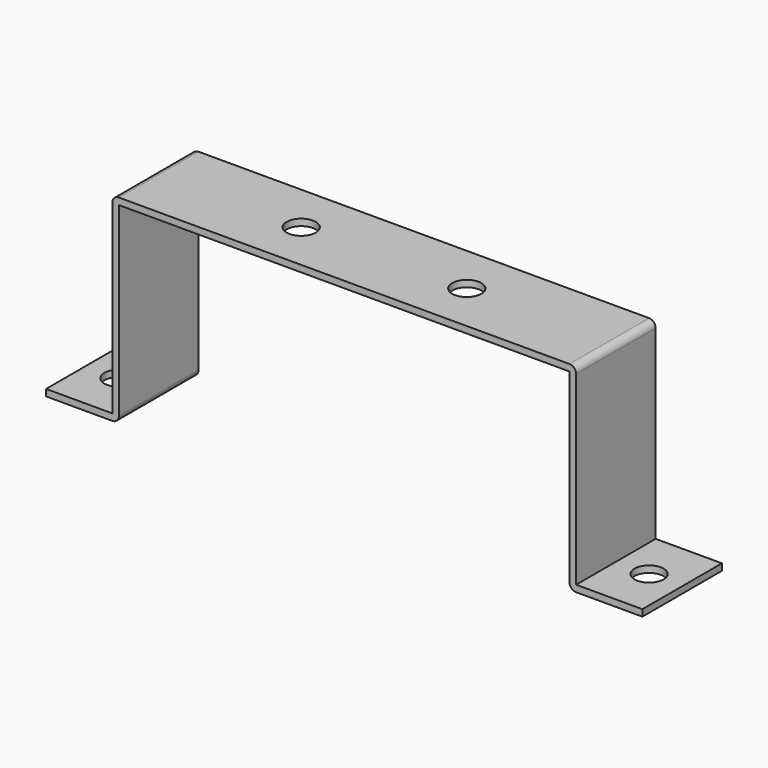
from build123d import *

# Parameters (mm, degrees)
F1_DEPTH = 30
F2_R     = 4.4
F3_R     = 4.4
F4_DEPTH = 25
F5_R     = 2
F6_R     = 2


# Not quite as in the source:
# - a feature names something its author has since deleted; it is built from what else it names


with BuildPart() as f1:
    # F0 (on Front) → F1 (new body)
    with BuildSketch(Plane.XZ):
        Polygon((90, -1), (90, 1), (70, 1), (70, 59), (-70, 59), (-70, 1), (-90, 1), (-90, -1), (-68, -1), (-68, 57), (68, 57), (68, -1), align=None)
    extrude(amount=F1_DEPTH)

    # F2 (on face) + F3 (on face) → F4 (cut)
    with BuildSketch(Plane.XY.offset(1)):
        with Locations((-80, -15)):
            Circle(F2_R)
        with Locations((80, -15)):
            Circle(F2_R)
    with BuildSketch(Plane.XY.offset(59)):
        with Locations((-25, -15)):
            Circle(F3_R)
        with Locations((25, -15)):
            Circle(F3_R)
    extrude(amount=-F4_DEPTH, mode=Mode.SUBTRACT)

    # F5
    f5_edges = [f1.edges().sort_by_distance(p)[0] for p in [
        (-70, -15, 59),
        (70, -15, 59),
    ]]
    fillet(f5_edges, radius=F5_R)

    # F6
    f6_edges = [f1.edges().sort_by_distance(p)[0] for p in [
        (68, -15, -1),
        (-68, -15, -1),
    ]]
    fillet(f6_edges, radius=F6_R)


solid = f1.part
